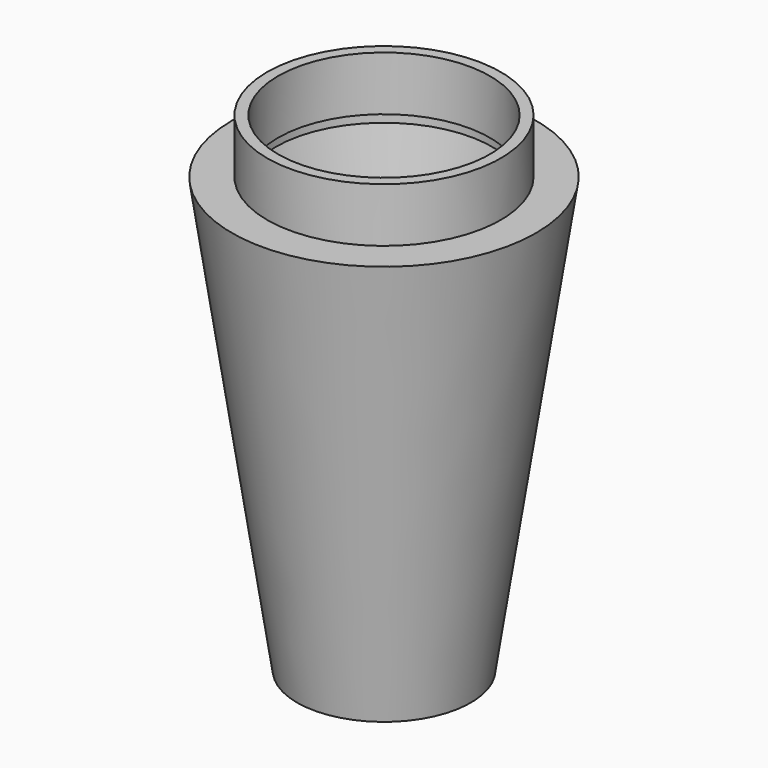
from build123d import *

# Parameters (mm, degrees)
F0_W = 3.175
F0_H = 15.875
F2_T = 2.54


# Not quite as in the source:
# - a shell that OpenCascade refuses in one call is made with other operations: the cavity is built on its own and cut out


with BuildPart() as f1:
    # F0 (on Front) → F1 (revolve)
    with BuildSketch(Plane.XZ):
        Polygon((0, -84.1329338265), (0, 42.8670661735), (-30.9626, 42.8670661735), (-34.1376, 42.8670661735), (-44.45, 42.8670661735), (-25.4, -84.1329338265), align=None)
        with Locations((-32.5501, 50.8045661735)):
            Rectangle(F0_W, F0_H)
    revolve(axis=Axis((0, 0, -17.2506261634), (0, 0, -1)))

    # F2: shell of thickness 2.54, made by hand


with BuildPart() as f2_core1:
    # F2_t2: copy of F1
    add(f1.part)

    # the walls: a layer under each face that stays
    f2_faces = [f2_core1.faces().sort_by_distance(p)[0] for p in [
        (30.9626, 0, 50.8045661735),
        (-22.7584, -22.7584, 58.7420661735),
        (34.1376, 0, 50.8045661735),
        (-29.6333333333, -29.6333333333, 42.8670661735),
        (34.925, 0, -20.6329338265),
        (0, 0, -84.1329338265),
    ]]
    thicken(f2_faces, amount=-F2_T, mode=Mode.SUBTRACT)

    # F2_s3 → F2_t4 (revolve, cut)
    with BuildSketch(Plane.XZ):
        Polygon((-34.163, 42.8924661735), (-31.5976, 42.8670661735), (-31.5976, 40.3270661735), (-34.1376, 40.3270661735), align=None)
    revolve(axis=Axis((0, 0, 42.8670661735), (0, 0, -1)), mode=Mode.SUBTRACT)


with BuildPart() as f1_1:
    add(f1.part)

    # what is left inside the walls is the cavity
    f2_cavity = [f2_core1.part.solids().sort_by_distance(p)[0] for p in [
        (35.379465, 0, -0.309166),
    ]]
    add(f2_cavity, mode=Mode.SUBTRACT)


solid = f1_1.part
